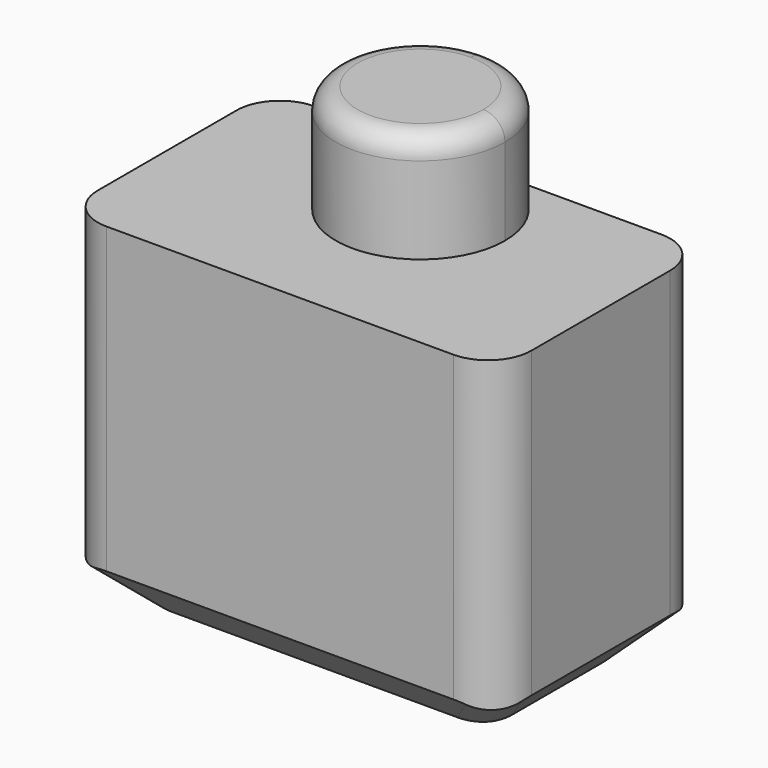
from build123d import *

# Parameters (mm, degrees)
F1_DEPTH = 8
F2_DEPTH = 2.5
F3_R     = 0.5
F4_SIZE  = 1
F5_F1_R  = 1
F5_F2_R  = 1
F5_F3_R  = 1
F5_F4_R  = 1
F5_F5_R  = 1
F5_F6_R  = 1
F5_F7_R  = 1
F5_F8_R  = 1


with BuildPart() as f1:
    # F0 (on Top) → F1 (new body)
    with BuildSketch(Plane.XY):
        Polygon((-5, -3), (5, -3), (5, 3), (0, 3), (-5, 3), align=None)
        with BuildLine():
            ThreePointArc((1.95, 1.05), (-1.3788582233, -0.3288582233), (0, 3))
            ThreePointArc((0, 3), (1.3788582233, 2.4288582233), (1.95, 1.05))
        make_face(mode=Mode.SUBTRACT)
        with BuildLine():
            ThreePointArc((1.95, 1.05), (1.3788582233, 2.4288582233), (0, 3))
            ThreePointArc((0, 3), (-1.3788582233, -0.3288582233), (1.95, 1.05))
        make_face()
    extrude(amount=-F1_DEPTH)

    # F0 (on Top) → F2 (join)
    with BuildSketch(Plane.XY):
        with BuildLine():
            ThreePointArc((1.95, 1.05), (1.3788582233, 2.4288582233), (0, 3))
            ThreePointArc((0, 3), (-1.3788582233, -0.3288582233), (1.95, 1.05))
        make_face()
    extrude(amount=F2_DEPTH)

    # F3
    f3_edges = [f1.edges().sort_by_distance(p)[0] for p in [
        (-1.95, 1.05, 2.5),
    ]]
    fillet(f3_edges, radius=F3_R)

    # F4
    f4_edges = [f1.edges().sort_by_distance(p)[0] for p in [
        (-5, 0, -8),
        (0, -3, -8),
        (0, 3, -8),
        (5, 0, -8),
    ]]
    chamfer(f4_edges, length=F4_SIZE)

    # F5: fillet of radius 1 on 8 edges, made by hand

    # F5_f1
    f5_f1_edges = [f1.edges().sort_by_distance(p)[0] for p in [
        (5, 3, -3.5),
    ]]
    fillet(f5_f1_edges, radius=F5_F1_R)

    # F5_f2
    f5_f2_edges = [f1.edges().sort_by_distance(p)[0] for p in [
        (-5, 3, -3.5),
    ]]
    fillet(f5_f2_edges, radius=F5_F2_R)

    # F5_f3
    f5_f3_edges = [f1.edges().sort_by_distance(p)[0] for p in [
        (5, -3, -3.5),
    ]]
    fillet(f5_f3_edges, radius=F5_F3_R)

    # F5_f4
    f5_f4_edges = [f1.edges().sort_by_distance(p)[0] for p in [
        (4.3535533906, 2.3535533906, -7.6464466094),
    ]]
    fillet(f5_f4_edges, radius=F5_F4_R)

    # F5_f5
    f5_f5_edges = [f1.edges().sort_by_distance(p)[0] for p in [
        (-4.3535533906, 2.3535533906, -7.6464466094),
    ]]
    fillet(f5_f5_edges, radius=F5_F5_R)

    # F5_f6
    f5_f6_edges = [f1.edges().sort_by_distance(p)[0] for p in [
        (-5, -3, -3.5),
    ]]
    fillet(f5_f6_edges, radius=F5_F6_R)

    # F5_f7
    f5_f7_edges = [f1.edges().sort_by_distance(p)[0] for p in [
        (4.3535533906, -2.3535533906, -7.6464466094),
    ]]
    fillet(f5_f7_edges, radius=F5_F7_R)

    # F5_f8
    f5_f8_edges = [f1.edges().sort_by_distance(p)[0] for p in [
        (-4.3535533906, -2.3535533906, -7.6464466094),
    ]]
    fillet(f5_f8_edges, radius=F5_F8_R)


solid = f1.part
